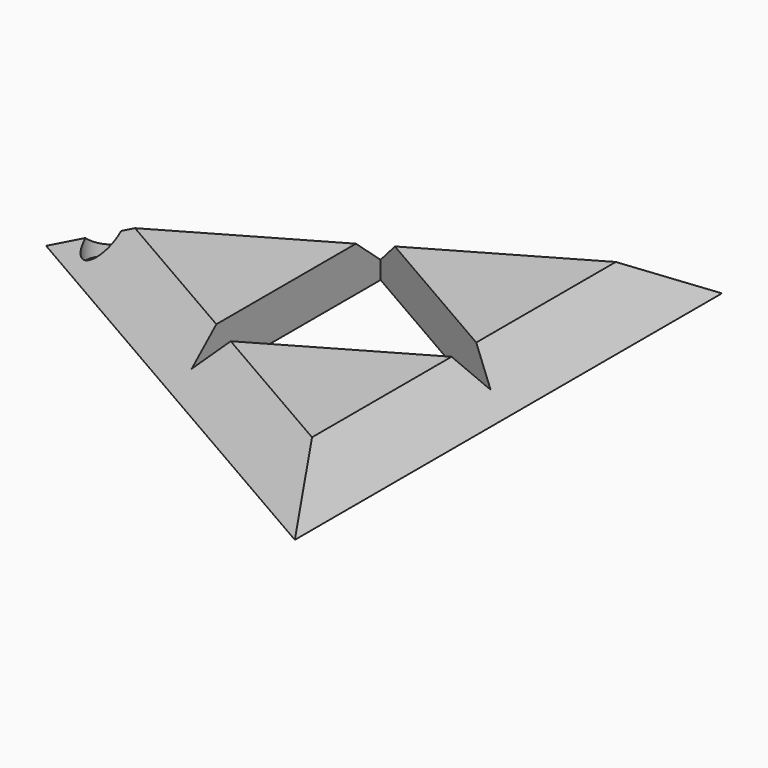
from build123d import *

# Parameters (mm, degrees)
F1_DEPTH    = 5
F2_R        = 2
F3_DEPTH    = 25
F4_T1_DEPTH = 85.7168298797
F4_T3_DEPTH = 85.7168298797
F4_T5_DEPTH = 85.7168298797


# Not quite as in the source:
# - a fillet or chamfer that OpenCascade refuses, or shapes differently, is made with other operations: its cross-section is extruded or revolved along the edge and cut away or added


with BuildPart() as f1:
    # F0 (on Top) → F1 (new body)
    with BuildSketch(Plane.XY):
        Polygon((17.3205080757, -30), (17.3205080757, 30), (-34.6410161514, 0), align=None)
        Polygon((-7.6602540378, -13.2679491924), (-7.6602540378, 13.2679491924), (15.3205080757, 0), align=None, mode=Mode.SUBTRACT)
    extrude(amount=F1_DEPTH)

    # F2 (on face) → F3 (cut)
    with BuildSketch(Plane.XY.offset(5)):
        with Locations((-28.2111279666, 0)):
            Circle(F2_R)
    extrude(amount=-F3_DEPTH, mode=Mode.SUBTRACT)

    # F4: chamfer of 5 on 3 edges, made by hand

    # F4_s2 → F4_t1 (cut)
    with BuildSketch(Plane(origin=(37.1164761038, 21.4292074699, 0), x_dir=(0, 0, 1), z_dir=(-0.8660254038, -0.5, 0))):
        Polygon((0, 17.3205080757), (5, 12.3205080757), (5, 17.3205080757), align=None)
    extrude(amount=F4_T1_DEPTH, mode=Mode.SUBTRACT)

    # F4_s4 → F4_t3 (cut)
    with BuildSketch(Plane.XZ.offset(-42.8584149398)):
        Polygon((17.3205080757, 0), (12.3205080757, 5), (17.3205080757, 5), align=None)
    extrude(amount=F4_T3_DEPTH, mode=Mode.SUBTRACT)

    # F4_s6 → F4_t5 (cut)
    with BuildSketch(Plane(origin=(-37.1164761038, 21.4292074699, 0), x_dir=(0, 0, 1), z_dir=(0.8660254038, -0.5, 0))):
        Polygon((0, 17.3205080757), (5, 12.3205080757), (5, 17.3205080757), align=None)
    extrude(amount=F4_T5_DEPTH, mode=Mode.SUBTRACT)


solid = f1.part
